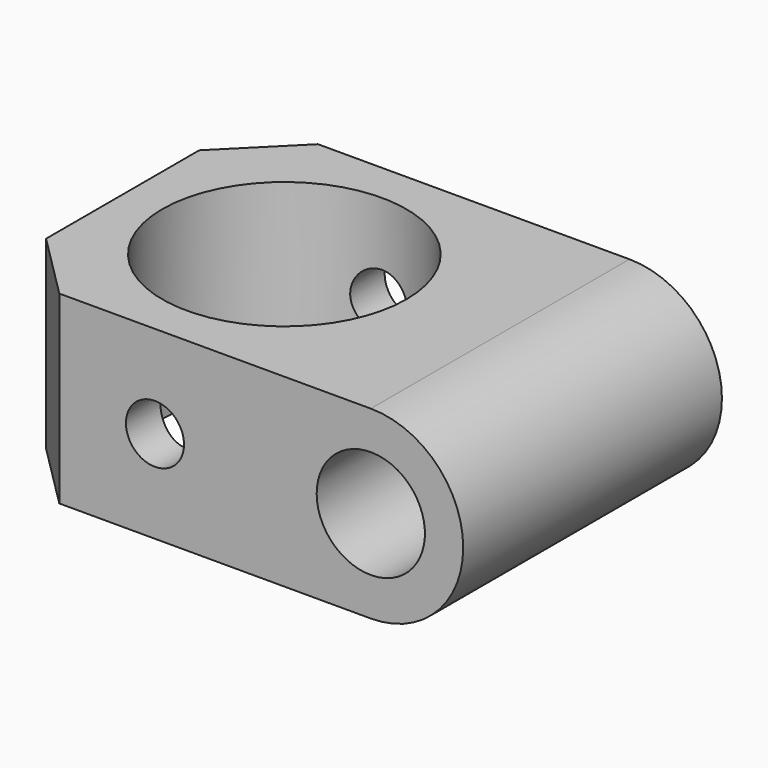
from build123d import *

# Parameters (mm, degrees)
F0_W     = 24.5
F0_H     = 24.5
F0_R     = 9.25
F1_DEPTH = 14
F2_R     = 2.2
F3_DEPTH = 24.5
F2_R_2   = 4.1
F4_DEPTH = 24.5
F5_START = -3
F5_DEPTH = 21.5
F6_SIZE  = 5


# Not quite as in the source:
# - a feature of the source that left no trace in its solid (it failed there, or was rolled back) is left out


with BuildPart() as f1:
    # F0 (on Top) → F1 (new body)
    with BuildSketch(Plane.XY):
        Rectangle(F0_W, F0_H)
        Circle(F0_R, mode=Mode.SUBTRACT)
    extrude(amount=F1_DEPTH)

    # F2 (on face) → F3 (cut, through all)
    with BuildSketch(Plane(origin=(0, 12.25, 0), x_dir=(-1, 0, 0), z_dir=(0, 1, 0))):
        with Locations((0, 7)):
            Circle(F2_R)
    extrude(amount=-F3_DEPTH, mode=Mode.SUBTRACT)

    # F2 (on face) → F4 (join, through all)
    with BuildSketch(Plane(origin=(0, 12.25, 0), x_dir=(-1, 0, 0), z_dir=(0, 1, 0))):
        with BuildLine():
            Line((-12.25, 7), (-12.25, 14))
            Line((-12.25, 14), (-16.35, 14))
            ThreePointArc((-16.35, 14), (-23.35, 7), (-16.35, 0))
            Line((-16.35, 0), (-12.25, 0))
            Line((-12.25, 0), (-12.25, 7))
        make_face()
        with Locations((-16.35, 7)):
            Circle(F2_R_2, mode=Mode.SUBTRACT)
        with Locations((-16.35, 7)):
            Circle(F2_R_2)
    extrude(amount=-F4_DEPTH)

    # F2 (on face) → F5 (cut)
    with BuildSketch(Plane(origin=(0, 12.25, 0), x_dir=(-1, 0, 0), z_dir=(0, 1, 0)).offset(F5_START)):
        with Locations((-16.35, 7)):
            Circle(F2_R_2)
    extrude(amount=-F5_DEPTH, mode=Mode.SUBTRACT)

    # F6
    f6_edges = [f1.edges().sort_by_distance(p)[0] for p in [
        (-12.25, 12.25, 7),
        (-12.25, -12.25, 7),
    ]]
    chamfer(f6_edges, length=F6_SIZE)


solid = f1.part
